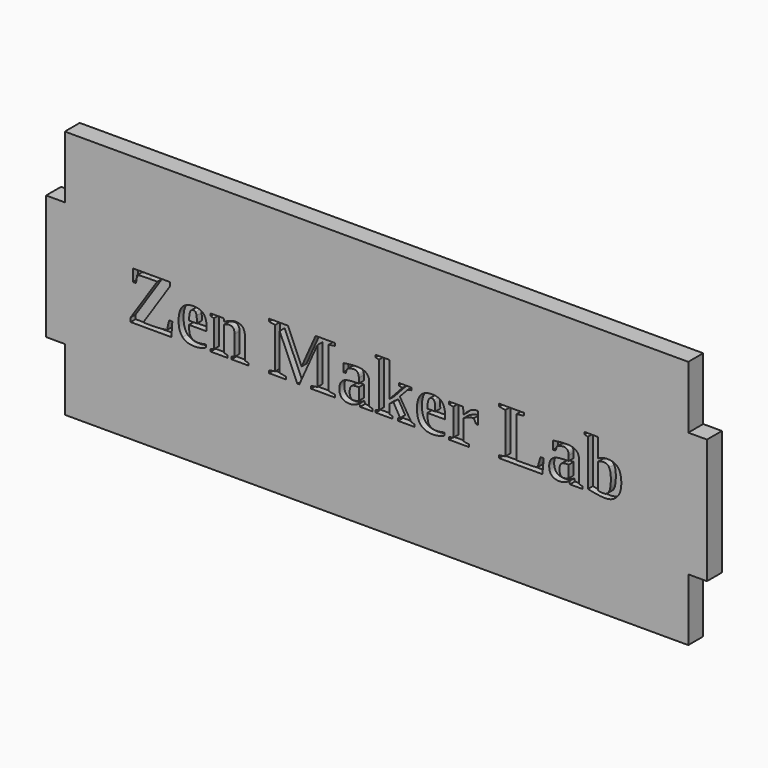
from build123d import *

# Parameters (mm, degrees)
F1_DEPTH     = 3
F0_TEXT_SIZE = 11.7647058824
F2_DEPTH     = 2


# Not quite as in the source:
# - Text() gives the source's letters only with a copy of the font that has no kerning and outlines rounded to 1/6400 em; it was checked with that copy


with BuildPart() as f1:
    # F0 (on Front) → F1 (new body)
    with BuildSketch(Plane.XZ):
        Polygon((50, 10), (50, 20), (-50, 20), (-50, 10), (-53, 10), (-53, -10), (-50, -10), (-50, -20), (50, -20), (50, -10), (53, -10), (53, 10), align=None)
        with BuildLine():
            add(Edge.make_bspline(
                [(-31.1443014706, 1.3658088235), (-30.5386029412, 2.0606617647), (-29.3143382353, 2.0606617647)],
                knots=[0, 0, 0, 1, 1, 1], degree=2))
            add(Edge.make_bspline(
                [(-29.3143382353, 2.0606617647), (-28.2169117647, 2.0606617647), (-27.7261029412, 1.4751838235)],
                knots=[0, 0, 0, 1, 1, 1], degree=2))
            add(Edge.make_bspline(
                [(-27.7261029412, 1.4751838235), (-27.2352941176, 0.8897058824), (-27.2352941176, -0.3455882353)],
                knots=[0, 0, 0, 1, 1, 1], degree=2))
            Line((-27.2352941176, -0.3455882353), (-27.2352941176, -0.8161764706))
            Line((-27.2352941176, -0.8161764706), (-30.0680147059, -0.8161764706))
            Line((-30.0680147059, -0.8161764706), (-30.0680147059, -0.9080882353))
            add(Edge.make_bspline(
                [(-30.0680147059, -0.9080882353), (-30.0680147059, -1.7647058824), (-29.9301470588, -2.1268382353)],
                knots=[0, 0, 0, 1, 1, 1], degree=2))
            add(Edge.make_bspline(
                [(-29.9301470588, -2.1268382353), (-29.7922794118, -2.4889705882), (-29.4816176471, -2.6783088235)],
                knots=[0, 0, 0, 1, 1, 1], degree=2))
            add(Edge.make_bspline(
                [(-29.4816176471, -2.6783088235), (-29.1709558824, -2.8676470588), (-28.6305147059, -2.8676470588)],
                knots=[0, 0, 0, 1, 1, 1], degree=2))
            add(Edge.make_bspline(
                [(-28.6305147059, -2.8676470588), (-28.125, -2.8676470588), (-27.3566176471, -2.7003676471)],
                knots=[0, 0, 0, 1, 1, 1], degree=2))
            Line((-27.3566176471, -2.7003676471), (-27.3566176471, -3.1433823529))
            add(Edge.make_bspline(
                [(-27.3566176471, -3.1433823529), (-27.6709558824, -3.3327205882), (-28.1737132353, -3.4558823529)],
                knots=[0, 0, 0, 1, 1, 1], degree=2))
            add(Edge.make_bspline(
                [(-28.1737132353, -3.4558823529), (-28.6764705882, -3.5790441176), (-29.1544117647, -3.5790441176)],
                knots=[0, 0, 0, 1, 1, 1], degree=2))
            add(Edge.make_bspline(
                [(-29.1544117647, -3.5790441176), (-30.4816176471, -3.5790441176), (-31.1158088235, -2.8869485294)],
                knots=[0, 0, 0, 1, 1, 1], degree=2))
            add(Edge.make_bspline(
                [(-31.1158088235, -2.8869485294), (-31.75, -2.1948529412), (-31.75, -0.7426470588)],
                knots=[0, 0, 0, 1, 1, 1], degree=2))
            add(Edge.make_bspline(
                [(-31.75, -0.7426470588), (-31.75, 0.6709558824), (-31.1443014706, 1.3658088235)],
                knots=[0, 0, 0, 1, 1, 1], degree=2))
        make_face(mode=Mode.SUBTRACT)
        with BuildLine():
            Line((-24.5165441176, 1.9301470588), (-24.4375, 1.4577205882))
            Line((-24.4375, 1.4577205882), (-24.0459558824, 1.6599264706))
            add(Edge.make_bspline(
                [(-24.0459558824, 1.6599264706), (-23.2426470588, 2.0735294118), (-22.5992647059, 2.0735294118)],
                knots=[0, 0, 0, 1, 1, 1], degree=2))
            add(Edge.make_bspline(
                [(-22.5992647059, 2.0735294118), (-21.1047794118, 2.0735294118), (-21.1047794118, 0.4816176471)],
                knots=[0, 0, 0, 1, 1, 1], degree=2))
            Line((-21.1047794118, 0.4816176471), (-21.1047794118, -2.9540441176))
            Line((-21.1047794118, -2.9540441176), (-20.5643382353, -3.0919117647))
            Line((-20.5643382353, -3.0919117647), (-20.5643382353, -3.4705882353))
            Line((-20.5643382353, -3.4705882353), (-23.2481617647, -3.4705882353))
            Line((-23.2481617647, -3.4705882353), (-23.2481617647, -3.0919117647))
            Line((-23.2481617647, -3.0919117647), (-22.7647058824, -2.9540441176))
            Line((-22.7647058824, -2.9540441176), (-22.7647058824, 0.2573529412))
            add(Edge.make_bspline(
                [(-22.7647058824, 0.2573529412), (-22.7647058824, 0.7408088235), (-22.96875, 1.0101102941)],
                knots=[0, 0, 0, 1, 1, 1], degree=2))
            add(Edge.make_bspline(
                [(-22.96875, 1.0101102941), (-23.1727941176, 1.2794117647), (-23.5514705882, 1.2794117647)],
                knots=[0, 0, 0, 1, 1, 1], degree=2))
            add(Edge.make_bspline(
                [(-23.5514705882, 1.2794117647), (-23.9889705882, 1.2794117647), (-24.4246323529, 1.0845588235)],
                knots=[0, 0, 0, 1, 1, 1], degree=2))
            Line((-24.4246323529, 1.0845588235), (-24.4246323529, -2.9540441176))
            Line((-24.4246323529, -2.9540441176), (-23.9319852941, -3.0919117647))
            Line((-23.9319852941, -3.0919117647), (-23.9319852941, -3.4705882353))
            Line((-23.9319852941, -3.4705882353), (-26.6139705882, -3.4705882353))
            Line((-26.6139705882, -3.4705882353), (-26.6139705882, -3.0919117647))
            Line((-26.6139705882, -3.0919117647), (-26.0863970588, -2.9540441176))
            Line((-26.0863970588, -2.9540441176), (-26.0863970588, 1.4117647059))
            Line((-26.0863970588, 1.4117647059), (-26.6139705882, 1.5496323529))
            Line((-26.6139705882, 1.5496323529), (-26.6139705882, 1.9301470588))
            Line((-26.6139705882, 1.9301470588), (-24.5165441176, 1.9301470588))
        make_face(mode=Mode.SUBTRACT)
        with BuildLine():
            add(Edge.make_bspline(
                [(-4.0386029412, 2.015625), (-3.6305147059, 2.0496323529), (-3.2058823529, 2.0496323529)],
                knots=[0, 0, 0, 1, 1, 1], degree=2))
            add(Edge.make_bspline(
                [(-3.2058823529, 2.0496323529), (-1.1783088235, 2.0496323529), (-1.1783088235, 0.5569852941)],
                knots=[0, 0, 0, 1, 1, 1], degree=2))
            Line((-1.1783088235, 0.5569852941), (-1.1783088235, -2.9540441176))
            Line((-1.1783088235, -2.9540441176), (-0.6378676471, -3.0919117647))
            Line((-0.6378676471, -3.0919117647), (-0.6378676471, -3.4705882353))
            Line((-0.6378676471, -3.4705882353), (-2.625, -3.4705882353))
            Line((-2.625, -3.4705882353), (-2.7518382353, -3.0569852941))
            add(Edge.make_bspline(
                [(-2.7518382353, -3.0569852941), (-3.2003676471, -3.3621323529), (-3.5615808824, -3.4742647059)],
                knots=[0, 0, 0, 1, 1, 1], degree=2))
            add(Edge.make_bspline(
                [(-3.5615808824, -3.4742647059), (-3.9227941176, -3.5863970588), (-4.2904411765, -3.5863970588)],
                knots=[0, 0, 0, 1, 1, 1], degree=2))
            add(Edge.make_bspline(
                [(-4.2904411765, -3.5863970588), (-5.9632352941, -3.5863970588), (-5.9632352941, -1.9761029412)],
                knots=[0, 0, 0, 1, 1, 1], degree=2))
            add(Edge.make_bspline(
                [(-5.9632352941, -1.9761029412), (-5.9632352941, -1.3676470588), (-5.7159926471, -1.0027573529)],
                knots=[0, 0, 0, 1, 1, 1], degree=2))
            add(Edge.make_bspline(
                [(-5.7159926471, -1.0027573529), (-5.46875, -0.6378676471), (-5.0036764706, -0.4632352941)],
                knots=[0, 0, 0, 1, 1, 1], degree=2))
            add(Edge.make_bspline(
                [(-5.0036764706, -0.4632352941), (-4.5386029412, -0.2886029412), (-3.5386029412, -0.2647058824)],
                knots=[0, 0, 0, 1, 1, 1], degree=2))
            Line((-3.5386029412, -0.2647058824), (-2.8382352941, -0.2481617647))
            Line((-2.8382352941, -0.2481617647), (-2.8382352941, 0.5386029412))
            add(Edge.make_bspline(
                [(-2.8382352941, 0.5386029412), (-2.8382352941, 1.5165441176), (-3.6360294118, 1.5165441176)],
                knots=[0, 0, 0, 1, 1, 1], degree=2))
            add(Edge.make_bspline(
                [(-3.6360294118, 1.5165441176), (-4.1194852941, 1.5165441176), (-4.7169117647, 1.2169117647)],
                knots=[0, 0, 0, 1, 1, 1], degree=2))
            Line((-4.7169117647, 1.2169117647), (-4.9338235294, 0.5441176471))
            Line((-4.9338235294, 0.5441176471), (-5.3143382353, 0.5441176471))
            Line((-5.3143382353, 0.5441176471), (-5.3143382353, 1.8492647059))
            add(Edge.make_bspline(
                [(-5.3143382353, 1.8492647059), (-4.4466911765, 1.9816176471), (-4.0386029412, 2.015625)],
                knots=[0, 0, 0, 1, 1, 1], degree=2))
        make_face(mode=Mode.SUBTRACT)
        with BuildLine():
            add(Edge.make_bspline(
                [(7.0909926471, 1.3658088235), (7.6966911765, 2.0606617647), (8.9209558824, 2.0606617647)],
                knots=[0, 0, 0, 1, 1, 1], degree=2))
            add(Edge.make_bspline(
                [(8.9209558824, 2.0606617647), (10.0183823529, 2.0606617647), (10.5091911765, 1.4751838235)],
                knots=[0, 0, 0, 1, 1, 1], degree=2))
            add(Edge.make_bspline(
                [(10.5091911765, 1.4751838235), (11, 0.8897058824), (11, -0.3455882353)],
                knots=[0, 0, 0, 1, 1, 1], degree=2))
            Line((11, -0.3455882353), (11, -0.8161764706))
            Line((11, -0.8161764706), (8.1672794118, -0.8161764706))
            Line((8.1672794118, -0.8161764706), (8.1672794118, -0.9080882353))
            add(Edge.make_bspline(
                [(8.1672794118, -0.9080882353), (8.1672794118, -1.7647058824), (8.3051470588, -2.1268382353)],
                knots=[0, 0, 0, 1, 1, 1], degree=2))
            add(Edge.make_bspline(
                [(8.3051470588, -2.1268382353), (8.4430147059, -2.4889705882), (8.7536764706, -2.6783088235)],
                knots=[0, 0, 0, 1, 1, 1], degree=2))
            add(Edge.make_bspline(
                [(8.7536764706, -2.6783088235), (9.0643382353, -2.8676470588), (9.6047794118, -2.8676470588)],
                knots=[0, 0, 0, 1, 1, 1], degree=2))
            add(Edge.make_bspline(
                [(9.6047794118, -2.8676470588), (10.1102941176, -2.8676470588), (10.8786764706, -2.7003676471)],
                knots=[0, 0, 0, 1, 1, 1], degree=2))
            Line((10.8786764706, -2.7003676471), (10.8786764706, -3.1433823529))
            add(Edge.make_bspline(
                [(10.8786764706, -3.1433823529), (10.5643382353, -3.3327205882), (10.0615808824, -3.4558823529)],
                knots=[0, 0, 0, 1, 1, 1], degree=2))
            add(Edge.make_bspline(
                [(10.0615808824, -3.4558823529), (9.5588235294, -3.5790441176), (9.0808823529, -3.5790441176)],
                knots=[0, 0, 0, 1, 1, 1], degree=2))
            add(Edge.make_bspline(
                [(9.0808823529, -3.5790441176), (7.7536764706, -3.5790441176), (7.1194852941, -2.8869485294)],
                knots=[0, 0, 0, 1, 1, 1], degree=2))
            add(Edge.make_bspline(
                [(7.1194852941, -2.8869485294), (6.4852941176, -2.1948529412), (6.4852941176, -0.7426470588)],
                knots=[0, 0, 0, 1, 1, 1], degree=2))
            add(Edge.make_bspline(
                [(6.4852941176, -0.7426470588), (6.4852941176, 0.6709558824), (7.0909926471, 1.3658088235)],
                knots=[0, 0, 0, 1, 1, 1], degree=2))
        make_face(mode=Mode.SUBTRACT)
        with BuildLine():
            Line((13.8897058824, 1.9301470588), (13.9540441176, 0.8088235294))
            add(Edge.make_bspline(
                [(13.9540441176, 0.8088235294), (14.5735294118, 1.4981617647), (15.0652573529, 1.7996323529)],
                knots=[0, 0, 0, 1, 1, 1], degree=2))
            add(Edge.make_bspline(
                [(15.0652573529, 1.7996323529), (15.5569852941, 2.1011029412), (15.9632352941, 2.1011029412)],
                knots=[0, 0, 0, 1, 1, 1], degree=2))
            Line((15.9632352941, 2.1011029412), (16.2738970588, 2.1011029412))
            Line((16.2738970588, 2.1011029412), (16.2738970588, 0.1305147059))
            Line((16.2738970588, 0.1305147059), (15.9522058824, 0.1305147059))
            Line((15.9522058824, 0.1305147059), (15.6139705882, 0.8547794118))
            add(Edge.make_bspline(
                [(15.6139705882, 0.8547794118), (15.2518382353, 0.8547794118), (14.7922794118, 0.6966911765)],
                knots=[0, 0, 0, 1, 1, 1], degree=2))
            add(Edge.make_bspline(
                [(14.7922794118, 0.6966911765), (14.3327205882, 0.5386029412), (13.9816176471, 0.3272058824)],
                knots=[0, 0, 0, 1, 1, 1], degree=2))
            Line((13.9816176471, 0.3272058824), (13.9816176471, -2.9540441176))
            Line((13.9816176471, -2.9540441176), (14.8492647059, -3.0919117647))
            Line((14.8492647059, -3.0919117647), (14.8492647059, -3.4705882353))
            Line((14.8492647059, -3.4705882353), (11.6213235294, -3.4705882353))
            Line((11.6213235294, -3.4705882353), (11.6213235294, -3.0919117647))
            Line((11.6213235294, -3.0919117647), (12.3216911765, -2.9540441176))
            Line((12.3216911765, -2.9540441176), (12.3216911765, 1.4117647059))
            Line((12.3216911765, 1.4117647059), (11.6213235294, 1.5496323529))
            Line((11.6213235294, 1.5496323529), (11.6213235294, 1.9301470588))
            Line((11.6213235294, 1.9301470588), (13.8897058824, 1.9301470588))
        make_face(mode=Mode.SUBTRACT)
        with BuildLine():
            add(Edge.make_bspline(
                [(29.6194852941, 2.015625), (30.0275735294, 2.0496323529), (30.4522058824, 2.0496323529)],
                knots=[0, 0, 0, 1, 1, 1], degree=2))
            add(Edge.make_bspline(
                [(30.4522058824, 2.0496323529), (32.4797794118, 2.0496323529), (32.4797794118, 0.5569852941)],
                knots=[0, 0, 0, 1, 1, 1], degree=2))
            Line((32.4797794118, 0.5569852941), (32.4797794118, -2.9540441176))
            Line((32.4797794118, -2.9540441176), (33.0202205882, -3.0919117647))
            Line((33.0202205882, -3.0919117647), (33.0202205882, -3.4705882353))
            Line((33.0202205882, -3.4705882353), (31.0330882353, -3.4705882353))
            Line((31.0330882353, -3.4705882353), (30.90625, -3.0569852941))
            add(Edge.make_bspline(
                [(30.90625, -3.0569852941), (30.4577205882, -3.3621323529), (30.0965073529, -3.4742647059)],
                knots=[0, 0, 0, 1, 1, 1], degree=2))
            add(Edge.make_bspline(
                [(30.0965073529, -3.4742647059), (29.7352941176, -3.5863970588), (29.3676470588, -3.5863970588)],
                knots=[0, 0, 0, 1, 1, 1], degree=2))
            add(Edge.make_bspline(
                [(29.3676470588, -3.5863970588), (27.6948529412, -3.5863970588), (27.6948529412, -1.9761029412)],
                knots=[0, 0, 0, 1, 1, 1], degree=2))
            add(Edge.make_bspline(
                [(27.6948529412, -1.9761029412), (27.6948529412, -1.3676470588), (27.9420955882, -1.0027573529)],
                knots=[0, 0, 0, 1, 1, 1], degree=2))
            add(Edge.make_bspline(
                [(27.9420955882, -1.0027573529), (28.1893382353, -0.6378676471), (28.6544117647, -0.4632352941)],
                knots=[0, 0, 0, 1, 1, 1], degree=2))
            add(Edge.make_bspline(
                [(28.6544117647, -0.4632352941), (29.1194852941, -0.2886029412), (30.1194852941, -0.2647058824)],
                knots=[0, 0, 0, 1, 1, 1], degree=2))
            Line((30.1194852941, -0.2647058824), (30.8198529412, -0.2481617647))
            Line((30.8198529412, -0.2481617647), (30.8198529412, 0.5386029412))
            add(Edge.make_bspline(
                [(30.8198529412, 0.5386029412), (30.8198529412, 1.5165441176), (30.0220588235, 1.5165441176)],
                knots=[0, 0, 0, 1, 1, 1], degree=2))
            add(Edge.make_bspline(
                [(30.0220588235, 1.5165441176), (29.5386029412, 1.5165441176), (28.9411764706, 1.2169117647)],
                knots=[0, 0, 0, 1, 1, 1], degree=2))
            Line((28.9411764706, 1.2169117647), (28.7242647059, 0.5441176471))
            Line((28.7242647059, 0.5441176471), (28.34375, 0.5441176471))
            Line((28.34375, 0.5441176471), (28.34375, 1.8492647059))
            add(Edge.make_bspline(
                [(28.34375, 1.8492647059), (29.2113970588, 1.9816176471), (29.6194852941, 2.015625)],
                knots=[0, 0, 0, 1, 1, 1], degree=2))
        make_face(mode=Mode.SUBTRACT)
        with BuildLine():
            Line((-39.4375, -3.4705882353), (-39.4375, -2.8161764706))
            Line((-39.4375, -2.8161764706), (-35.1746323529, 3.6231617647))
            Line((-35.1746323529, 3.6231617647), (-36.5533088235, 3.6231617647))
            add(Edge.make_bspline(
                [(-36.5533088235, 3.6231617647), (-37.8566176471, 3.6231617647), (-38.3915441176, 3.5091911765)],
                knots=[0, 0, 0, 1, 1, 1], degree=2))
            Line((-38.3915441176, 3.5091911765), (-38.5698529412, 2.2977941176))
            Line((-38.5698529412, 2.2977941176), (-39.0808823529, 2.2977941176))
            Line((-39.0808823529, 2.2977941176), (-39.0808823529, 4.2334558824))
            Line((-39.0808823529, 4.2334558824), (-33.1286764706, 4.2334558824))
            Line((-33.1286764706, 4.2334558824), (-33.1286764706, 3.6231617647))
            Line((-33.1286764706, 3.6231617647), (-37.4209558824, -2.8731617647))
            Line((-37.4209558824, -2.8731617647), (-35.8125, -2.8731617647))
            add(Edge.make_bspline(
                [(-35.8125, -2.8731617647), (-35.1580882353, -2.8731617647), (-34.5229779412, -2.8097426471)],
                knots=[0, 0, 0, 1, 1, 1], degree=2))
            add(Edge.make_bspline(
                [(-34.5229779412, -2.8097426471), (-33.8878676471, -2.7463235294), (-33.6066176471, -2.6838235294)],
                knots=[0, 0, 0, 1, 1, 1], degree=2))
            Line((-33.6066176471, -2.6838235294), (-33.2665441176, -1.2132352941))
            Line((-33.2665441176, -1.2132352941), (-32.75, -1.2132352941))
            Line((-32.75, -1.2132352941), (-32.90625, -3.4705882353))
            Line((-32.90625, -3.4705882353), (-39.4375, -3.4705882353))
        make_face(mode=Mode.SUBTRACT)
        Polygon((-9.4797794118, 3.0386029412), (-12.3805147059, -3.4705882353), (-12.6966911765, -3.4705882353), (-15.5386029412, 3.0386029412), (-15.5386029412, -2.8952205882), (-14.5055147059, -3.0514705882), (-14.5055147059, -3.4705882353), (-17.2463235294, -3.4705882353), (-17.2463235294, -3.0514705882), (-16.2573529412, -2.8952205882), (-16.2573529412, 3.6636029412), (-17.2463235294, 3.8143382353), (-17.2463235294, 4.2334558824), (-14.21875, 4.2334558824), (-12.0183823529, -0.8345588235), (-9.7720588235, 4.2334558824), (-6.6819852941, 4.2334558824), (-6.6819852941, 3.8143382353), (-7.6691176471, 3.6636029412), (-7.6691176471, -2.8952205882), (-6.6819852941, -3.0514705882), (-6.6819852941, -3.4705882353), (-10.5128676471, -3.4705882353), (-10.5128676471, -3.0514705882), (-9.4797794118, -2.8952205882), align=None, mode=Mode.SUBTRACT)
        Polygon((2.0459558824, 4.6930147059), (2.0459558824, -0.8805147059), (4.1525735294, 1.4172794118), (3.5790441176, 1.5496323529), (3.5790441176, 1.9301470588), (5.6360294118, 1.9301470588), (5.6360294118, 1.5496323529), (5.0147058824, 1.4246323529), (3.7279411765, 0.0680147059), (5.5845588235, -2.9540441176), (6.0661764706, -3.0919117647), (6.0661764706, -3.4705882353), (3.4705882353, -3.4705882353), (3.4705882353, -3.0919117647), (3.7849264706, -2.9540441176), (2.7058823529, -1.0643382353), (2.0459558824, -1.5238970588), (2.0459558824, -2.9540441176), (2.5790441176, -3.0919117647), (2.5790441176, -3.4705882353), (-0.1268382353, -3.4705882353), (-0.1268382353, -3.0919117647), (0.3841911765, -2.9540441176), (0.3841911765, 4.1746323529), (-0.1672794118, 4.3125), (-0.1672794118, 4.6930147059), align=None, mode=Mode.SUBTRACT)
        with BuildLine():
            Line((23.65625, 4.2334558824), (23.65625, 3.8143382353))
            Line((23.65625, 3.8143382353), (22.4669117647, 3.6636029412))
            Line((22.4669117647, 3.6636029412), (22.4669117647, -2.8621323529))
            Line((22.4669117647, -2.8621323529), (24.0349264706, -2.8621323529))
            add(Edge.make_bspline(
                [(24.0349264706, -2.8621323529), (25.2591911765, -2.8621323529), (25.8345588235, -2.7463235294)],
                knots=[0, 0, 0, 1, 1, 1], degree=2))
            Line((25.8345588235, -2.7463235294), (26.3051470588, -1.1433823529))
            Line((26.3051470588, -1.1433823529), (26.8216911765, -1.1433823529))
            Line((26.8216911765, -1.1433823529), (26.6029411765, -3.4705882353))
            Line((26.6029411765, -3.4705882353), (19.6691176471, -3.4705882353))
            Line((19.6691176471, -3.4705882353), (19.6691176471, -3.0514705882))
            Line((19.6691176471, -3.0514705882), (20.6580882353, -2.8952205882))
            Line((20.6580882353, -2.8952205882), (20.6580882353, 3.6636029412))
            Line((20.6580882353, 3.6636029412), (19.6764705882, 3.8143382353))
            Line((19.6764705882, 3.8143382353), (19.6764705882, 4.2334558824))
            Line((19.6764705882, 4.2334558824), (23.65625, 4.2334558824))
        make_face(mode=Mode.SUBTRACT)
        with BuildLine():
            Line((33.8988970588, -3.1948529412), (33.8988970588, 4.1875))
            Line((33.8988970588, 4.1875), (33.3474264706, 4.3198529412))
            Line((33.3474264706, 4.3198529412), (33.3474264706, 4.6930147059))
            Line((33.3474264706, 4.6930147059), (35.5588235294, 4.6930147059))
            Line((35.5588235294, 4.6930147059), (35.5588235294, 2.7113970588))
            add(Edge.make_bspline(
                [(35.5588235294, 2.7113970588), (35.5588235294, 2.1764705882), (35.5018382353, 1.625)],
                knots=[0, 0, 0, 1, 1, 1], degree=2))
            add(Edge.make_bspline(
                [(35.5018382353, 1.625), (35.7316176471, 1.8143382353), (36.1654411765, 1.9439338235)],
                knots=[0, 0, 0, 1, 1, 1], degree=2))
            add(Edge.make_bspline(
                [(36.1654411765, 1.9439338235), (36.5992647059, 2.0735294118), (37.0128676471, 2.0735294118)],
                knots=[0, 0, 0, 1, 1, 1], degree=2))
            add(Edge.make_bspline(
                [(37.0128676471, 2.0735294118), (38.1856617647, 2.0735294118), (38.7251838235, 1.4301470588)],
                knots=[0, 0, 0, 1, 1, 1], degree=2))
            add(Edge.make_bspline(
                [(38.7251838235, 1.4301470588), (39.2647058824, 0.7867647059), (39.2647058824, -0.6213235294)],
                knots=[0, 0, 0, 1, 1, 1], degree=2))
            add(Edge.make_bspline(
                [(39.2647058824, -0.6213235294), (39.2647058824, -2.0110294118), (38.5726102941, -2.7987132353)],
                knots=[0, 0, 0, 1, 1, 1], degree=2))
            add(Edge.make_bspline(
                [(38.5726102941, -2.7987132353), (37.8805147059, -3.5863970588), (36.6231617647, -3.5863970588)],
                knots=[0, 0, 0, 1, 1, 1], degree=2))
            add(Edge.make_bspline(
                [(36.6231617647, -3.5863970588), (35.6911764706, -3.5863970588), (33.8988970588, -3.1948529412)],
                knots=[0, 0, 0, 1, 1, 1], degree=2))
        make_face(mode=Mode.SUBTRACT)
    extrude(amount=F1_DEPTH)



with BuildPart() as f1b:
    # F0 (on Front) → F1, piece 2 (new body)
    with BuildSketch(Plane.XZ):
        with BuildLine():
            add(Edge.make_bspline(
                [(-29.0358455882, 1.3318014706), (-29.1599264706, 1.4816176471), (-29.3786764706, 1.4816176471)],
                knots=[0, 0, 0, 1, 1, 1], degree=2))
            add(Edge.make_bspline(
                [(-29.3786764706, 1.4816176471), (-29.7224264706, 1.4816176471), (-29.8915441176, 1.1084558824)],
                knots=[0, 0, 0, 1, 1, 1], degree=2))
            add(Edge.make_bspline(
                [(-29.8915441176, 1.1084558824), (-30.0606617647, 0.7352941176), (-30.0606617647, -0.2132352941)],
                knots=[0, 0, 0, 1, 1, 1], degree=2))
            Line((-30.0606617647, -0.2132352941), (-28.8088235294, -0.2132352941))
            add(Edge.make_bspline(
                [(-28.8088235294, -0.2132352941), (-28.8088235294, 0.5569852941), (-28.8602941176, 0.8694852941)],
                knots=[0, 0, 0, 1, 1, 1], degree=2))
            add(Edge.make_bspline(
                [(-28.8602941176, 0.8694852941), (-28.9117647059, 1.1819852941), (-29.0358455882, 1.3318014706)],
                knots=[0, 0, 0, 1, 1, 1], degree=2))
        make_face()
    extrude(amount=F1_DEPTH)


with BuildPart() as f1c:
    # F0 (on Front) → F1, piece 3 (new body)
    with BuildSketch(Plane.XZ):
        with BuildLine():
            Line((-2.8382352941, -2.6893382353), (-2.8382352941, -0.7591911765))
            Line((-2.8382352941, -0.7591911765), (-3.3198529412, -0.7757352941))
            add(Edge.make_bspline(
                [(-3.3198529412, -0.7757352941), (-3.8768382353, -0.7996323529), (-4.0928308824, -1.0698529412)],
                knots=[0, 0, 0, 1, 1, 1], degree=2))
            add(Edge.make_bspline(
                [(-4.0928308824, -1.0698529412), (-4.3088235294, -1.3400735294), (-4.3088235294, -1.9430147059)],
                knots=[0, 0, 0, 1, 1, 1], degree=2))
            add(Edge.make_bspline(
                [(-4.3088235294, -1.9430147059), (-4.3088235294, -2.4301470588), (-4.1360294118, -2.6599264706)],
                knots=[0, 0, 0, 1, 1, 1], degree=2))
            add(Edge.make_bspline(
                [(-4.1360294118, -2.6599264706), (-3.9632352941, -2.8897058824), (-3.6875, -2.8897058824)],
                knots=[0, 0, 0, 1, 1, 1], degree=2))
            add(Edge.make_bspline(
                [(-3.6875, -2.8897058824), (-3.2977941176, -2.8897058824), (-2.8382352941, -2.6893382353)],
                knots=[0, 0, 0, 1, 1, 1], degree=2))
        make_face()
    extrude(amount=F1_DEPTH)


with BuildPart() as f1d:
    # F0 (on Front) → F1, piece 4 (new body)
    with BuildSketch(Plane.XZ):
        with BuildLine():
            add(Edge.make_bspline(
                [(9.1994485294, 1.3318014706), (9.0753676471, 1.4816176471), (8.8566176471, 1.4816176471)],
                knots=[0, 0, 0, 1, 1, 1], degree=2))
            add(Edge.make_bspline(
                [(8.8566176471, 1.4816176471), (8.5128676471, 1.4816176471), (8.34375, 1.1084558824)],
                knots=[0, 0, 0, 1, 1, 1], degree=2))
            add(Edge.make_bspline(
                [(8.34375, 1.1084558824), (8.1746323529, 0.7352941176), (8.1746323529, -0.2132352941)],
                knots=[0, 0, 0, 1, 1, 1], degree=2))
            Line((8.1746323529, -0.2132352941), (9.4264705882, -0.2132352941))
            add(Edge.make_bspline(
                [(9.4264705882, -0.2132352941), (9.4264705882, 0.5569852941), (9.375, 0.8694852941)],
                knots=[0, 0, 0, 1, 1, 1], degree=2))
            add(Edge.make_bspline(
                [(9.375, 0.8694852941), (9.3235294118, 1.1819852941), (9.1994485294, 1.3318014706)],
                knots=[0, 0, 0, 1, 1, 1], degree=2))
        make_face()
    extrude(amount=F1_DEPTH)


with BuildPart() as f1e:
    # F0 (on Front) → F1, piece 5 (new body)
    with BuildSketch(Plane.XZ):
        with BuildLine():
            Line((30.8198529412, -2.6893382353), (30.8198529412, -0.7591911765))
            Line((30.8198529412, -0.7591911765), (30.3382352941, -0.7757352941))
            add(Edge.make_bspline(
                [(30.3382352941, -0.7757352941), (29.78125, -0.7996323529), (29.5652573529, -1.0698529412)],
                knots=[0, 0, 0, 1, 1, 1], degree=2))
            add(Edge.make_bspline(
                [(29.5652573529, -1.0698529412), (29.3492647059, -1.3400735294), (29.3492647059, -1.9430147059)],
                knots=[0, 0, 0, 1, 1, 1], degree=2))
            add(Edge.make_bspline(
                [(29.3492647059, -1.9430147059), (29.3492647059, -2.4301470588), (29.5220588235, -2.6599264706)],
                knots=[0, 0, 0, 1, 1, 1], degree=2))
            add(Edge.make_bspline(
                [(29.5220588235, -2.6599264706), (29.6948529412, -2.8897058824), (29.9705882353, -2.8897058824)],
                knots=[0, 0, 0, 1, 1, 1], degree=2))
            add(Edge.make_bspline(
                [(29.9705882353, -2.8897058824), (30.3602941176, -2.8897058824), (30.8198529412, -2.6893382353)],
                knots=[0, 0, 0, 1, 1, 1], degree=2))
        make_face()
    extrude(amount=F1_DEPTH)


with BuildPart() as f1f:
    # F0 (on Front) → F1, piece 6 (new body)
    with BuildSketch(Plane.XZ):
        with BuildLine():
            add(Edge.make_bspline(
                [(37.3051470588, -2.4273897059), (37.5808823529, -1.8731617647), (37.5808823529, -0.6158088235)],
                knots=[0, 0, 0, 1, 1, 1], degree=2))
            add(Edge.make_bspline(
                [(37.5808823529, -0.6158088235), (37.5808823529, 0.4466911765), (37.3198529412, 0.9411764706)],
                knots=[0, 0, 0, 1, 1, 1], degree=2))
            add(Edge.make_bspline(
                [(37.3198529412, 0.9411764706), (37.0588235294, 1.4356617647), (36.4613970588, 1.4356617647)],
                knots=[0, 0, 0, 1, 1, 1], degree=2))
            add(Edge.make_bspline(
                [(36.4613970588, 1.4356617647), (36.2426470588, 1.4356617647), (35.984375, 1.3869485294)],
                knots=[0, 0, 0, 1, 1, 1], degree=2))
            add(Edge.make_bspline(
                [(35.984375, 1.3869485294), (35.7261029412, 1.3382352941), (35.5588235294, 1.2408088235)],
                knots=[0, 0, 0, 1, 1, 1], degree=2))
            Line((35.5588235294, 1.2408088235), (35.5588235294, -2.8897058824))
            add(Edge.make_bspline(
                [(35.5588235294, -2.8897058824), (35.9264705882, -2.9816176471), (36.4613970588, -2.9816176471)],
                knots=[0, 0, 0, 1, 1, 1], degree=2))
            add(Edge.make_bspline(
                [(36.4613970588, -2.9816176471), (37.0294117647, -2.9816176471), (37.3051470588, -2.4273897059)],
                knots=[0, 0, 0, 1, 1, 1], degree=2))
        make_face()
    extrude(amount=F1_DEPTH)


with BuildPart() as f1_1:
    add(f1.part)

    add(f1b.part)  # F2 merges F1b

    add(f1c.part)  # F2 merges F1c

    add(f1d.part)  # F2 merges F1d

    add(f1e.part)  # F2 merges F1e

    add(f1f.part)  # F2 merges F1f
    # F0 (on Front) → F2 (join)
    with BuildSketch(Plane.XZ):
        with Locations((-40, -3.4705882353)):
            Text('Zen Maker Lab', F0_TEXT_SIZE, font='Tinos', font_style=FontStyle.BOLD, text_align=(TextAlign.LEFT, TextAlign.BOTTOM))
    extrude(amount=F2_DEPTH)


solid = f1_1.part
